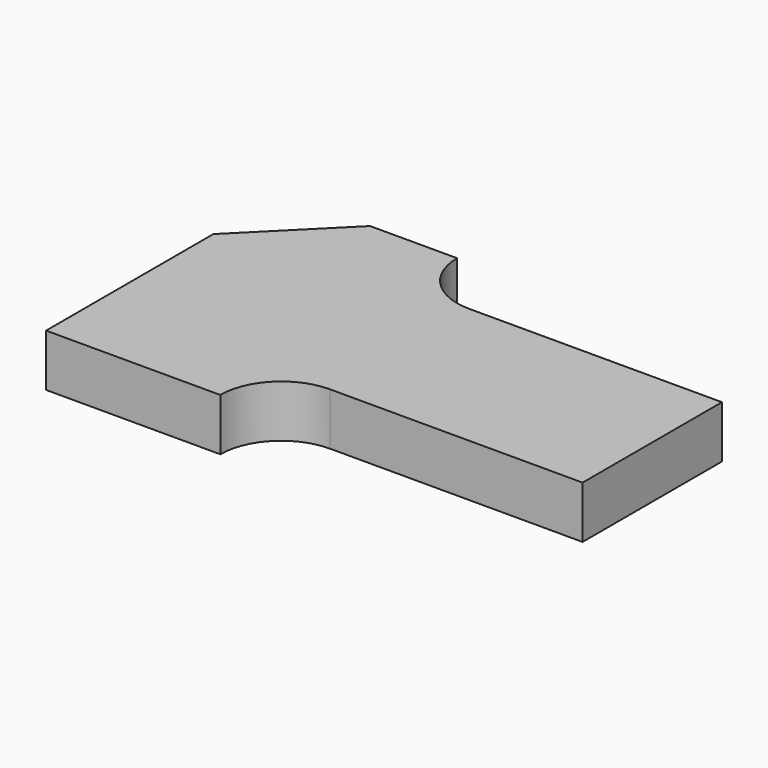
from build123d import *

# Parameters (mm, degrees)
F1_DEPTH = 3
F2_R     = 3.49999
F3_R     = 3.49999


# Not quite as in the source:
# - a fillet or chamfer is up to 0.001 mm smaller than in the source, because OpenCascade refuses the exact size


with BuildPart() as f1:
    # F0 (on Top) → F1 (new body)
    with BuildSketch(Plane.XY):
        Polygon((0, 12), (0, 0), (10, 0), (10, 3.5), (28, 3.5), (28, 13.5), (10, 13.5), (10, 17), (5, 17), align=None)
    extrude(amount=F1_DEPTH)

    # F2 (radius 3.5 in the source; OpenCascade refuses exactly that, so slightly less here)
    f2_edges = [f1.edges().sort_by_distance(p)[0] for p in [
        (10, 13.5, 1.5),
    ]]
    fillet(f2_edges, radius=F2_R)

    # F3 (radius 3.5 in the source; OpenCascade refuses exactly that, so slightly less here)
    f3_edges = [f1.edges().sort_by_distance(p)[0] for p in [
        (10, 3.5, 1.5),
    ]]
    fillet(f3_edges, radius=F3_R)


solid = f1.part
